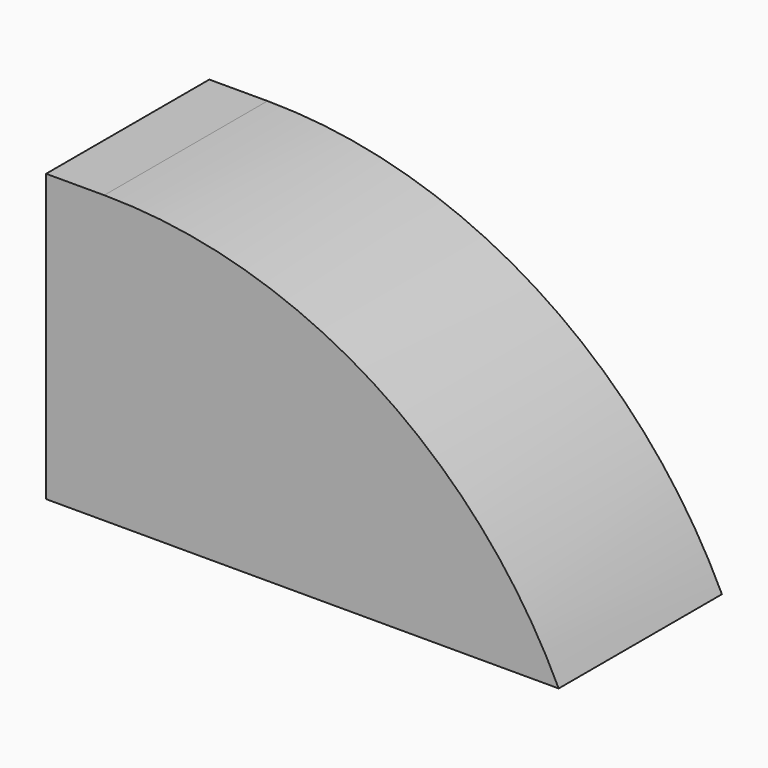
from build123d import *

# Parameters (mm, degrees)
F0_W        = 144.9560448527
F0_H        = 57.6972393319
F1_DEPTH    = 81
F2_T1_DEPTH = 700.2323206536


# Not quite as in the source:
# - a fillet or chamfer that OpenCascade refuses, or shapes differently, is made with other operations: its cross-section is extruded or revolved along the edge and cut away or added


with BuildPart() as f1:
    # F0 (on Top) → F1 (new body)
    with BuildSketch(Plane.XY):
        with Locations((-30.1226638258, -35.9269068576)):
            Rectangle(F0_W, F0_H)
    extrude(amount=F1_DEPTH)

    # F2: fillet of radius 142.43860018 on 1 edges, made by hand

    # F2_s2 → F2_t1 (cut)
    with BuildSketch(Plane.XZ.offset(-314.1892534691)):
        with BuildLine():
            ThreePointArc((42.3553586006, 0), (-10.199282406, 59.060327259), (-86.1516576637, 81))
            Line((-86.1516576637, 81), (42.3553586006, 81))
            Line((42.3553586006, 81), (42.3553586006, 0))
        make_face()
    extrude(amount=F2_T1_DEPTH, mode=Mode.SUBTRACT)


solid = f1.part
